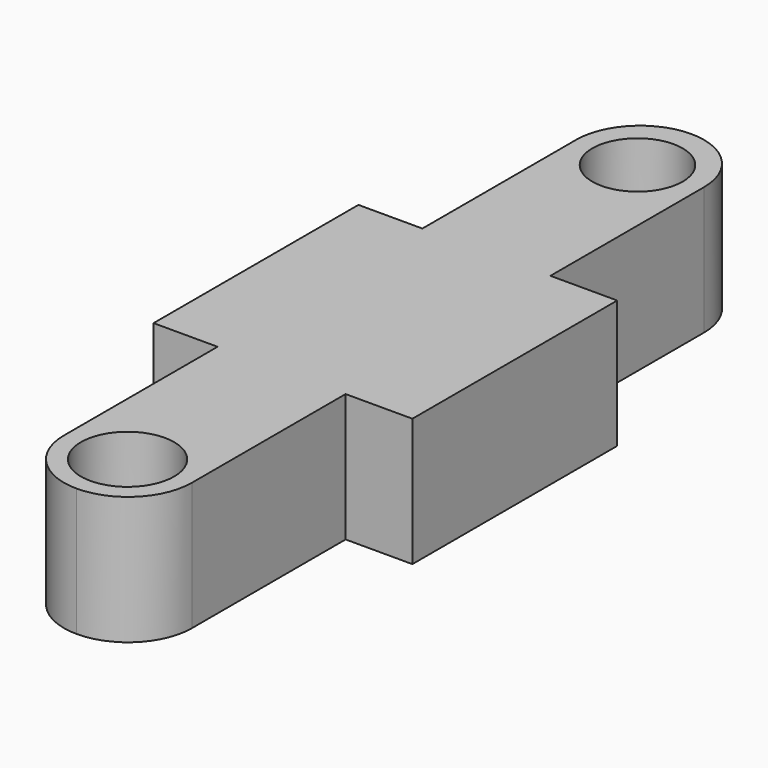
from build123d import *

# Parameters (mm, degrees)
F0_R     = 7.2809687116
F0_R_2   = 7.0556428797
F1_DEPTH = 20
F2_R     = 9.99999


# Not quite as in the source:
# - a fillet or chamfer is up to 0.001 mm smaller than in the source, because OpenCascade refuses the exact size


with BuildPart() as f1:
    # F0 (on Top) → F1 (new body)
    with BuildSketch(Plane.XY):
        Polygon((-20, 20), (-20, 0), (-20, -20), (-10, -20), (-10, -60), (10, -60), (10, -20), (20.4342082143, -20), (20.4342082143, 20), (10, 20), (10, 60), (-10, 60), (-10, 20), align=None)
        with Locations((0, -50.0781983137)):
            Circle(F0_R, mode=Mode.SUBTRACT)
        with Locations((0, 49.5025888085)):
            Circle(F0_R_2, mode=Mode.SUBTRACT)
    extrude(amount=F1_DEPTH)

    # F2 (radius 10 in the source; OpenCascade refuses exactly that, so slightly less here)
    f2_edges = [f1.edges().sort_by_distance(p)[0] for p in [
        (10, 60, 10),
        (-10, 60, 10),
        (10, -60, 10),
        (-10, -60, 10),
    ]]
    fillet(f2_edges, radius=F2_R)


solid = f1.part
